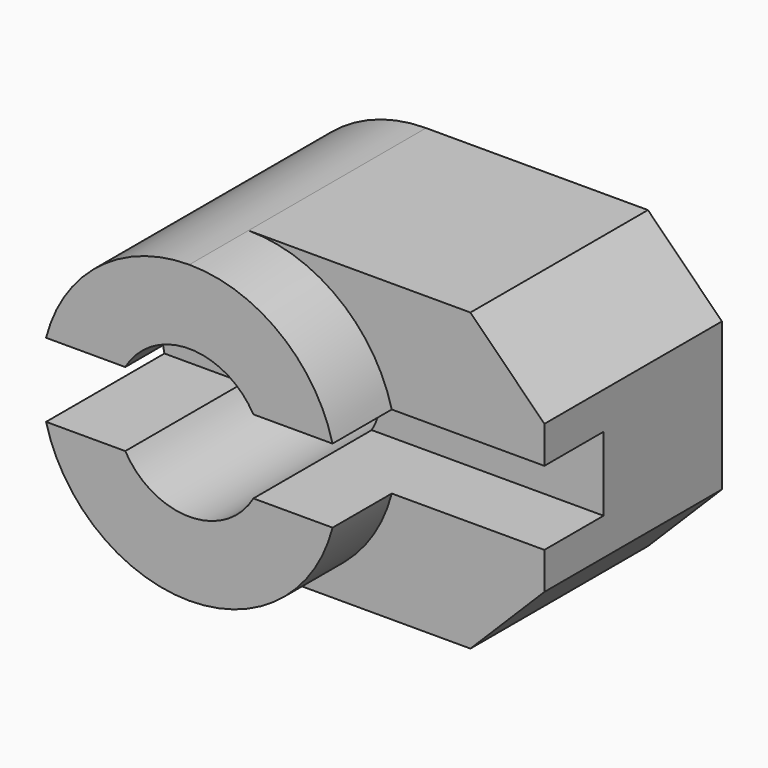
from build123d import *

# Parameters (mm, degrees)
F1_DEPTH = 20
F2_DEPTH = 10
F3_DEPTH = 15


with BuildPart() as f1:
    # F0 (on Front) → F1 (new body)
    with BuildSketch(Plane.XZ):
        with BuildLine():
            ThreePointArc((9.6824583655, 2.5), (6.123724357, 7.9056941504), (0, 10))
            ThreePointArc((0, 10), (-6.123724357, 7.9056941504), (-9.6824583655, 2.5))
            Line((-9.6824583655, 2.5), (-4.3301270189, 2.5))
            ThreePointArc((-4.3301270189, 2.5), (0, 5), (4.3301270189, 2.5))
            Line((4.3301270189, 2.5), (9.6824583655, 2.5))
        make_face()
    extrude(amount=F1_DEPTH)



with BuildPart() as f1b:
    # F0 (on Front) → F1, piece 2 (new body)
    with BuildSketch(Plane.XZ):
        with BuildLine():
            Line((-4.3301270189, -2.5), (-9.6824583655, -2.5))
            ThreePointArc((-9.6824583655, -2.5), (-6.123724357, -7.9056941504), (0, -10))
            ThreePointArc((0, -10), (6.123724357, -7.9056941504), (9.6824583655, -2.5))
            Line((9.6824583655, -2.5), (4.3301270189, -2.5))
            ThreePointArc((4.3301270189, -2.5), (0, -5), (-4.3301270189, -2.5))
        make_face()
    extrude(amount=F1_DEPTH)


with BuildPart() as f1_1:
    add(f1.part)

    add(f1b.part)  # F2 merges F1b
    # F0 (on Front) → F2 (join)
    with BuildSketch(Plane.XZ):
        with BuildLine():
            Line((20, 2.5), (9.6824583655, 2.5))
            ThreePointArc((9.6824583655, 2.5), (9.9202969627, 1.2600429248), (10, 0))
            ThreePointArc((10, 0), (9.9202969627, -1.2600429248), (9.6824583655, -2.5))
            Line((9.6824583655, -2.5), (20, -2.5))
            Line((20, -2.5), (20, 0))
            Line((20, 0), (20, 2.5))
        make_face()
        with BuildLine():
            ThreePointArc((10, 0), (9.9202969627, 1.2600429248), (9.6824583655, 2.5))
            Line((9.6824583655, 2.5), (4.3301270189, 2.5))
            ThreePointArc((4.3301270189, 2.5), (4.8296291314, 1.2940952255), (5, 0))
            ThreePointArc((5, 0), (4.8296291314, -1.2940952255), (4.3301270189, -2.5))
            Line((4.3301270189, -2.5), (9.6824583655, -2.5))
            ThreePointArc((9.6824583655, -2.5), (9.9202969627, -1.2600429248), (10, 0))
        make_face()
        with BuildLine():
            Line((-4.3301270189, 2.5), (-9.6824583655, 2.5))
            ThreePointArc((-9.6824583655, 2.5), (-10, 0), (-9.6824583655, -2.5))
            Line((-9.6824583655, -2.5), (-4.3301270189, -2.5))
            ThreePointArc((-4.3301270189, -2.5), (-5, 0), (-4.3301270189, 2.5))
        make_face()
    extrude(amount=F2_DEPTH)

    # F0 (on Front) → F3 (join)
    with BuildSketch(Plane.XZ):
        with BuildLine():
            Line((15, 10), (0, 10))
            ThreePointArc((0, 10), (6.123724357, 7.9056941504), (9.6824583655, 2.5))
            Line((9.6824583655, 2.5), (20, 2.5))
            Line((20, 2.5), (20, 5))
            Line((20, 5), (15, 10))
        make_face()
        with BuildLine():
            ThreePointArc((9.6824583655, -2.5), (6.123724357, -7.9056941504), (0, -10))
            Line((0, -10), (15, -10))
            Line((15, -10), (20, -5))
            Line((20, -5), (20, -2.5))
            Line((20, -2.5), (9.6824583655, -2.5))
        make_face()
    extrude(amount=F3_DEPTH)


solid = f1_1.part
